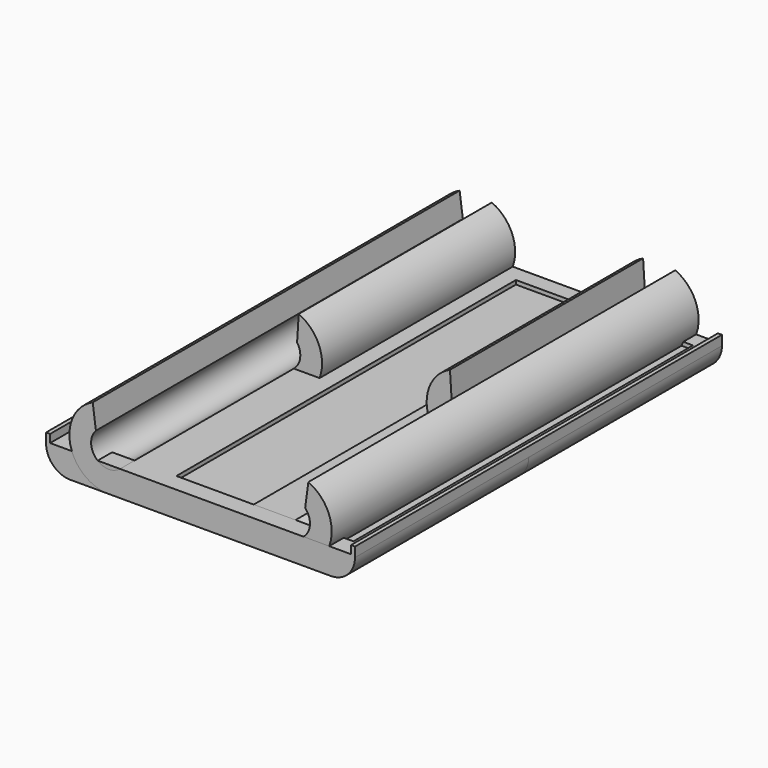
from build123d import *

# Parameters (mm, degrees)
F1_DEPTH = 30
F2_R     = 3
F4_DEPTH = 27
F5_W     = 22
F5_H     = 52.7442957759
F6_DEPTH = 0.5
F0_W     = 0.5
F0_H     = 1
F7_DEPTH = 57


# Not quite as in the source:
# - a feature names something its author has since deleted; it is built from what else it names


with BuildPart() as f1:
    # F0 (on Front) → F1 (new body)
    with BuildSketch(Plane.XZ):
        with BuildLine():
            Line((-18.695979941, 1.1248678452), (-19.195979941, 1.1248678452))
            Line((-19.195979941, 1.1248678452), (-19.195979941, -2.0751321548))
            Line((-19.195979941, -2.0751321548), (11.3996701762, -2.0751321548))
            ThreePointArc((11.3996701762, -2.0751321548), (16.1917962107, 1.8023571757), (13.3996701762, 7.2981216945))
            Line((13.3996701762, 7.2981216945), (13.0025328865, 4.3317955581))
            ThreePointArc((13.0025328865, 4.3317955581), (11.5532638802, 0.6302359913), (9.6025328865, 4.0938428497))
            Line((9.6025328865, 4.0938428497), (9.3996701762, 7.2981216945))
            ThreePointArc((9.3996701762, 7.2981216945), (6.8827114771, 4.724100351), (6.804020059, 1.1248678452))
            Line((6.804020059, 1.1248678452), (-18.695979941, 1.1248678452))
        make_face()
    extrude(amount=F1_DEPTH)

    # F2
    f2_edges = [f1.edges().sort_by_distance(p)[0] for p in [
        (-19.19598, -15, -2.075132),
    ]]
    fillet(f2_edges, radius=F2_R)

    # F3 (on face) → F4 (join)
    with BuildSketch(Plane.XZ.offset(30)):
        with BuildLine():
            Line((10.0032461718, 1.1248678452), (6.804020059, 1.1248678452))
            Line((6.804020059, 1.1248678452), (-19.195979941, 1.1248678452))
            Line((-19.195979941, 1.1248678452), (-19.195979941, 0.9248678452))
            ThreePointArc((-19.195979941, 0.9248678452), (-18.3173002846, -1.1964524984), (-16.195979941, -2.0751321548))
            Line((-16.195979941, -2.0751321548), (11.3996701762, -2.0751321548))
            ThreePointArc((11.3996701762, -2.0751321548), (16.1917962107, 1.8023571757), (13.3996701762, 7.2981216945))
            Line((13.3996701762, 7.2981216945), (13.0025328865, 4.3317955581))
            ThreePointArc((13.0025328865, 4.3317955581), (13.006452854, 1.3221205523), (10.0032461718, 1.1248678452))
        make_face()
    extrude(amount=F4_DEPTH)

    # F5 (on face) → F6 (cut)
    with BuildSketch(Plane.XY.offset(1.1248678452)):
        with Locations((-6.195979941, -28.3721478879)):
            Rectangle(F5_W, F5_H)
    extrude(amount=-F6_DEPTH, mode=Mode.SUBTRACT)

    # F0 (on Front) → F7 (join)
    with BuildSketch(Plane.XZ):
        with Locations((-18.945979941, 1.6248678452)):
            Rectangle(F0_W, F0_H)
    extrude(amount=F7_DEPTH)


with BuildPart() as f8_1:
    # F8: instance of F1
    add(f1.part.mirror(Plane.YZ))


solid = Compound([f1.part, f8_1.part])
